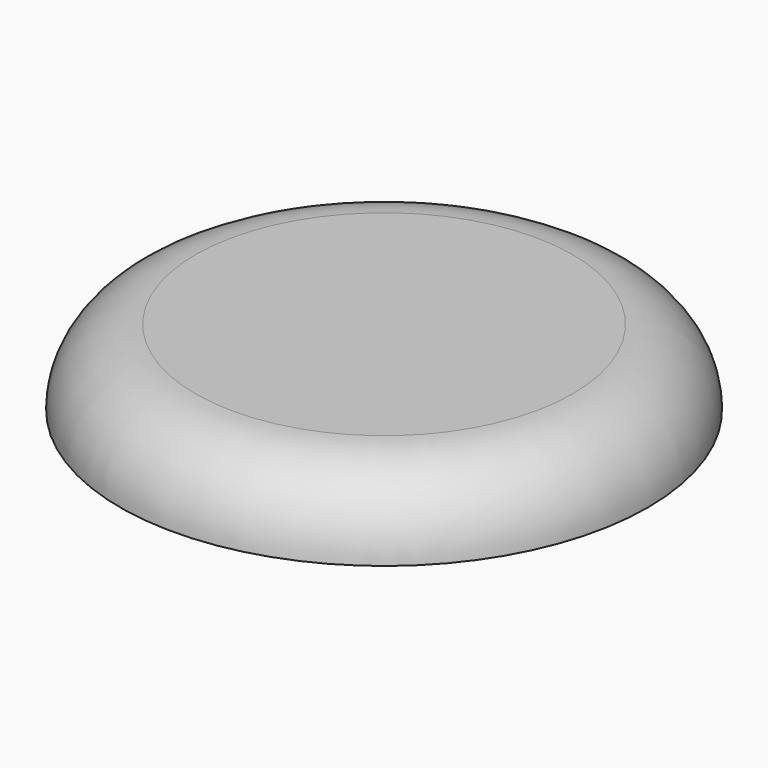
from build123d import *

# Parameters (mm, degrees)
F0_R     = 22.225
F1_DEPTH = 3.175
F2_R     = 6.34999


# Not quite as in the source:
# - a fillet or chamfer is up to 0.001 mm smaller than in the source, because OpenCascade refuses the exact size


with BuildPart() as f1:
    # F0 (on Top) → F1 (new body, symmetric)
    with BuildSketch(Plane.XY):
        Circle(F0_R)
    extrude(amount=F1_DEPTH, both=True)

    # F2 (radius 6.35 in the source; OpenCascade refuses exactly that, so slightly less here)
    f2_edges = [f1.edges().sort_by_distance(p)[0] for p in [
        (-22.225, 0, 3.175),
    ]]
    fillet(f2_edges, radius=F2_R)


solid = f1.part
